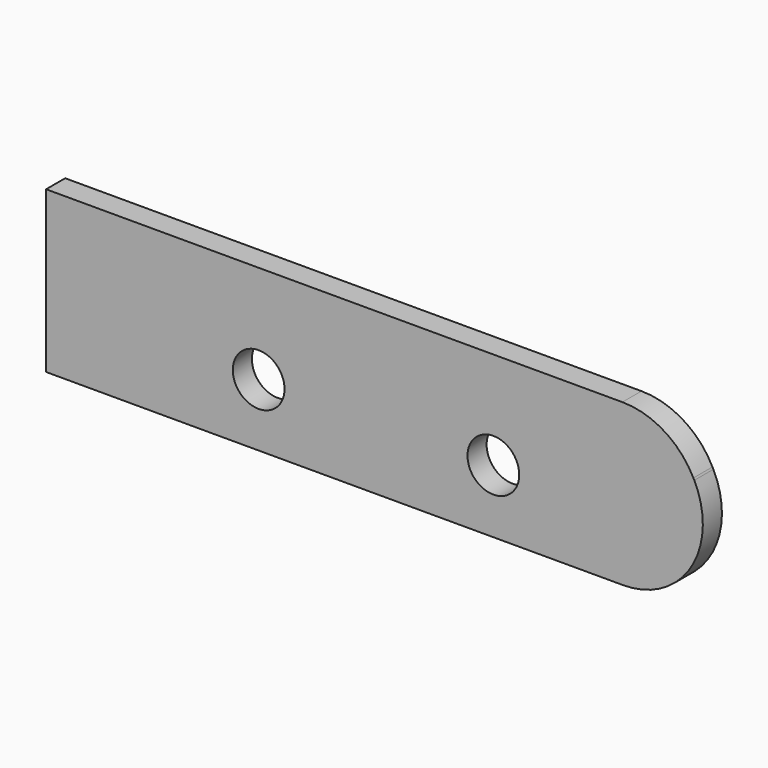
from build123d import *

# Parameters (mm, degrees)
F1_DEPTH       = 3
F3_D           = 3.3
F3_DEPTH       = 14.4
F3_CBORE_D     = 6.5
F3_CBORE_DEPTH = 3
F3_TIP         = 0.9914200214


# Not quite as in the source:
# - a feature names something its author has since deleted; it is built from what else it names


with BuildPart() as f1:
    # F0 (on Front) → F1 (new body)
    with BuildSketch(Plane.XZ):
        with BuildLine():
            Line((52.4541210128, 6.1781848239), (-19.9804399163, 6.1781848239))
            Line((-19.9804399163, 6.1781848239), (-19.9804399163, -14.0438194092))
            Line((-19.9804399163, -14.0438194092), (52.5663935712, -14.0438194092))
            ThreePointArc((52.5663935712, -14.0438194092), (61.0848860922, -9.2816896986), (61.4901453485, 0.469123557))
            Line((61.4901453485, 0.469123557), (61.3778727901, 0.6911277901))
            ThreePointArc((61.3778727901, 0.6911277901), (57.6919913022, 4.696677345), (52.4541210128, 6.1781848239))
        make_face()
    extrude(amount=F1_DEPTH)

    # F3
    with Locations(Plane.XZ.offset(3)):
        with Locations((36.2392867059, -6.078066061), (6.7392867059, -6.1909663491)):
            CounterBoreHole(F3_D / 2, F3_CBORE_D / 2, F3_CBORE_DEPTH, depth=F3_DEPTH)
            with Locations((0, 0, -(F3_DEPTH + F3_TIP / 2))):  # 118° drill point
                Cone(0, F3_D / 2, F3_TIP, mode=Mode.SUBTRACT)


solid = f1.part
